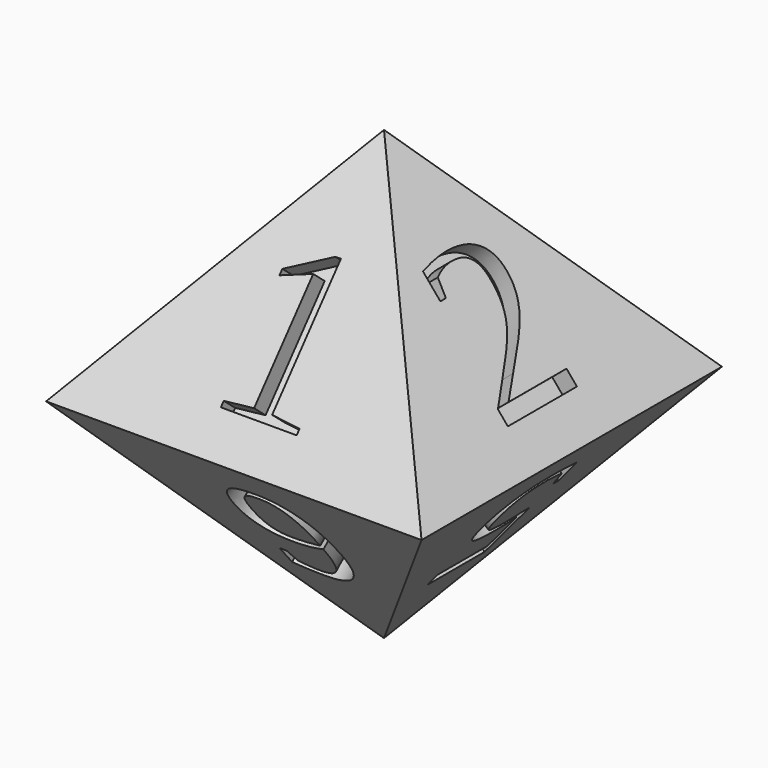
from build123d import *

# Parameters (mm, degrees)
F0_W          = 50.8
F0_H          = 50.8
F1_DEPTH      = 38.1
F1_TAPER      = 40
F3_TEXT_SIZE  = 29.1349442117
F4_DEPTH      = 2.54
F5_TEXT_SIZE  = 29.1349442117
F6_DEPTH      = 2.54
F7_TEXT_SIZE  = 29.1349442117
F8_DEPTH      = 2.54
F9_TEXT_SIZE  = 29.1349442117
F10_DEPTH     = 2.54
F11_TEXT_SIZE = 29.1349442117
F12_DEPTH     = 2.54
F13_TEXT_SIZE = 29.1349442117
F14_DEPTH     = 2.54
F15_TEXT_SIZE = 29.1349442117
F16_DEPTH     = 2.54
F17_TEXT_SIZE = 29.1349442117
F18_DEPTH     = 2.54


# Not quite as in the source:
# - an extrude whose draft closes it to a point is written as a loft to that point
# - Text() gives the source's letters only with a copy of the font that has no kerning and outlines rounded to 1/6400 em; it was checked with that copy


with BuildPart() as f1:
    # F0 (on Top) → F1 (new body)
    with BuildSketch(Plane.XY):
        Rectangle(F0_W, F0_H)
    extrude(amount=F1_DEPTH, taper=F1_TAPER)

    # F0 (on Top) → F2 section 0
    with BuildSketch(Plane.XY, mode=Mode.PRIVATE) as f2_s0:
        Rectangle(F0_W, F0_H)
    loft([f2_s0.sketch, Vertex(0, 0, -30.2705412519)], ruled=True)

    # F3 (on face) → F4 (cut)
    with BuildSketch(Plane(origin=(0, -14.9053318564, 12.5070584633), x_dir=(1, 0, 0), z_dir=(0, -0.7660444431, 0.6427876097))):
        with Locations((-7.3201547332, -10.4885799162)):
            Text('1', F3_TEXT_SIZE, font='Tinos', text_align=(TextAlign.LEFT, TextAlign.BOTTOM))
    extrude(amount=-F4_DEPTH, mode=Mode.SUBTRACT)

    # F5 (on face) → F6 (cut)
    with BuildSketch(Plane(origin=(0, 14.9053318564, -12.5070584633), x_dir=(-1, 0, 0), z_dir=(0, 0.7660444431, -0.6427876097))):
        with Locations(Location((7.6388181855, 10.4885799162), (0, 0, 180))):
            Text('8', F5_TEXT_SIZE, font='Tinos', text_align=(TextAlign.LEFT, TextAlign.BOTTOM))
    extrude(amount=-F6_DEPTH, mode=Mode.SUBTRACT)

    # F7 (on face) → F8 (cut)
    with BuildSketch(Plane(origin=(14.9053318564, 0, 12.5070584633), x_dir=(0, 1, 0), z_dir=(0.7660444431, 0, 0.6427876097))):
        with Locations((-7.3907159262, -10.4885799162)):
            Text('2', F7_TEXT_SIZE, font='Tinos', text_align=(TextAlign.LEFT, TextAlign.BOTTOM))
    extrude(amount=-F8_DEPTH, mode=Mode.SUBTRACT)

    # F9 (on face) → F10 (cut)
    with BuildSketch(Plane(origin=(-14.9053318564, 0, -12.5070584633), x_dir=(0, -1, 0), z_dir=(-0.7660444431, 0, -0.6427876097))):
        with Locations(Location((8.5333520195, 10.4885799162), (0, 0, 180))):
            Text('7', F9_TEXT_SIZE, font='Open Sans', text_align=(TextAlign.LEFT, TextAlign.BOTTOM))
    extrude(amount=-F10_DEPTH, mode=Mode.SUBTRACT)

    # F11 (on face) → F12 (cut)
    with BuildSketch(Plane(origin=(0, -14.9053318564, -12.5070584633), x_dir=(1, 0, 0), z_dir=(0, -0.7660444431, -0.6427876097))):
        with Locations(Location((7.7594550639, 10.4885799162), (0, 0, 180))):
            Text('6', F11_TEXT_SIZE, font='Tinos', text_align=(TextAlign.LEFT, TextAlign.BOTTOM))
    extrude(amount=-F12_DEPTH, mode=Mode.SUBTRACT)

    # F13 (on face) → F14 (cut)
    with BuildSketch(Plane(origin=(0, 14.9053318564, 12.5070584633), x_dir=(-1, 0, 0), z_dir=(0, 0.7660444431, 0.6427876097))):
        with Locations((-7.6251611804, -10.4885799162)):
            Text('3', F13_TEXT_SIZE, font='Tinos', text_align=(TextAlign.LEFT, TextAlign.BOTTOM))
    extrude(amount=-F14_DEPTH, mode=Mode.SUBTRACT)

    # F15 (on face) → F16 (cut)
    with BuildSketch(Plane(origin=(14.9053318564, 0, -12.5070584633), x_dir=(0, 1, 0), z_dir=(0.7660444431, 0, -0.6427876097))):
        with Locations(Location((7.6251611804, 10.4885799162), (0, 0, 180))):
            Text('5', F15_TEXT_SIZE, font='Tinos', text_align=(TextAlign.LEFT, TextAlign.BOTTOM))
    extrude(amount=-F16_DEPTH, mode=Mode.SUBTRACT)

    # F17 (on face) → F18 (cut)
    with BuildSketch(Plane(origin=(-14.9053318564, 0, 12.5070584633), x_dir=(0, -1, 0), z_dir=(-0.7660444431, 0, 0.6427876097))):
        with Locations((-7.9665863079, -10.4885799162)):
            Text('4', F17_TEXT_SIZE, font='Tinos', text_align=(TextAlign.LEFT, TextAlign.BOTTOM))
    extrude(amount=-F18_DEPTH, mode=Mode.SUBTRACT)


solid = f1.part
